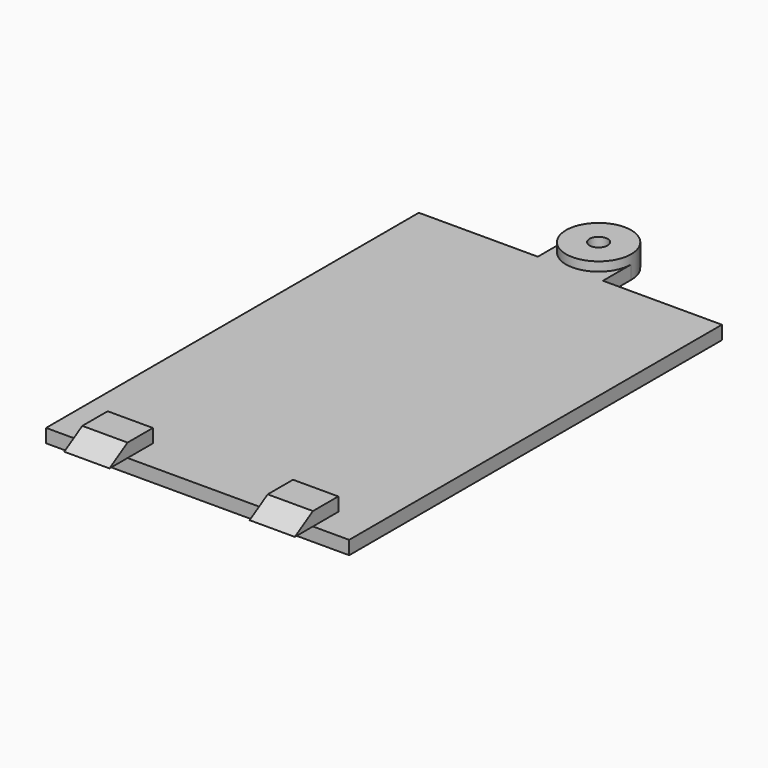
from build123d import *

# Parameters (mm, degrees)
F0_R     = 2
F0_R_2   = 1
F1_DEPTH = 1.5
F2_DEPTH = 2.5
F3_W     = 5
F3_H     = 2.5
F3_H_2   = 3.5
F4_DEPTH = 1.5
F5_SIZE2 = 2.49999
F5_SIZE  = 1.49999
F6_SIZE2 = 1.49999
F6_SIZE  = 2.49999
F7_DEPTH = 25
F8_DEPTH = 1


# Not quite as in the source:
# - a fillet or chamfer is up to 0.001 mm smaller than in the source, because OpenCascade refuses the exact size
# - a feature names something its author has since deleted; it is built from what else it names


with BuildPart() as f1:
    # F0 (on Top) → F1 (new body)
    with BuildSketch(Plane.XY):
        Polygon((-16.75, 0), (0, 0), (16.75, 0), (16.75, 51.5), (3.6, 51.5), (0, 51.5), (-3.6, 51.5), (-16.75, 51.5), align=None)
        with BuildLine():
            ThreePointArc((3.6, 55.4), (0, 59), (-3.6, 55.4))
            ThreePointArc((-3.6, 55.4), (0, 51.8), (3.6, 55.4))
        make_face()
        with Locations((0, 55.4)):
            Circle(F0_R, mode=Mode.SUBTRACT)
        with Locations((0, 55.4)):
            Circle(F0_R)
        with Locations((0, 55.4)):
            Circle(F0_R_2, mode=Mode.SUBTRACT)
        with BuildLine():
            Line((-3.6, 55.4), (-3.6, 51.5))
            Line((-3.6, 51.5), (0, 51.5))
            Line((0, 51.5), (3.6, 51.5))
            Line((3.6, 51.5), (3.6, 55.4))
            ThreePointArc((3.6, 55.4), (0, 51.8), (-3.6, 55.4))
        make_face()
        with Locations((0, 55.4)):
            Circle(F0_R_2)
    extrude(amount=F1_DEPTH)

    # F0 (on Top) → F2 (join)
    with BuildSketch(Plane.XY):
        with BuildLine():
            ThreePointArc((3.6, 55.4), (0, 59), (-3.6, 55.4))
            ThreePointArc((-3.6, 55.4), (0, 51.8), (3.6, 55.4))
        make_face()
        with Locations((0, 55.4)):
            Circle(F0_R, mode=Mode.SUBTRACT)
        with Locations((0, 55.4)):
            Circle(F0_R)
        with Locations((0, 55.4)):
            Circle(F0_R_2, mode=Mode.SUBTRACT)
        with Locations((0, 55.4)):
            Circle(F0_R_2)
    extrude(amount=F2_DEPTH)

    # F3 (on face) → F4 (join)
    with BuildSketch(Plane.XY.offset(1.5)):
        with Locations((-10.2441851608, -1.25)):
            Rectangle(F3_W, F3_H)
        with Locations((-10.2441851608, 1.75)):
            Rectangle(F3_W, F3_H_2)
        with Locations((10.2441851608, -1.25)):
            Rectangle(F3_W, F3_H)
        with Locations((10.2441851608, 1.75)):
            Rectangle(F3_W, F3_H_2)
    extrude(amount=F4_DEPTH)

    # F5 (size 1.5 and 2.5 in the source; OpenCascade refuses exactly that, so slightly less here)
    f5_edges = [f1.edges().sort_by_distance(p)[0] for p in [
        (-10.244185, -2.5, 3),
    ]]
    f5_side = f1.faces().sort_by_distance((-10.244185, -2.5, 2.25))[0]
    chamfer(f5_edges, length=F5_SIZE, length2=F5_SIZE2, reference=f5_side)

    # F6 (size 2.5 and 1.5 in the source; OpenCascade refuses exactly that, so slightly less here)
    f6_edges = [f1.edges().sort_by_distance(p)[0] for p in [
        (10.244185, -2.5, 3),
    ]]
    f6_side = f1.faces().sort_by_distance((10.244185, 0.5, 3))[0]
    chamfer(f6_edges, length=F6_SIZE, length2=F6_SIZE2, reference=f6_side)

    # F0 (on Top) → F7 (cut)
    with BuildSketch(Plane.XY):
        with Locations((0, 55.4)):
            Circle(F0_R_2)
    extrude(amount=F7_DEPTH, mode=Mode.SUBTRACT)

    # F0 (on Top) → F8 (cut)
    with BuildSketch(Plane.XY):
        with Locations((0, 55.4)):
            Circle(F0_R)
        with Locations((0, 55.4)):
            Circle(F0_R_2, mode=Mode.SUBTRACT)
    extrude(amount=F8_DEPTH, mode=Mode.SUBTRACT)


solid = f1.part
